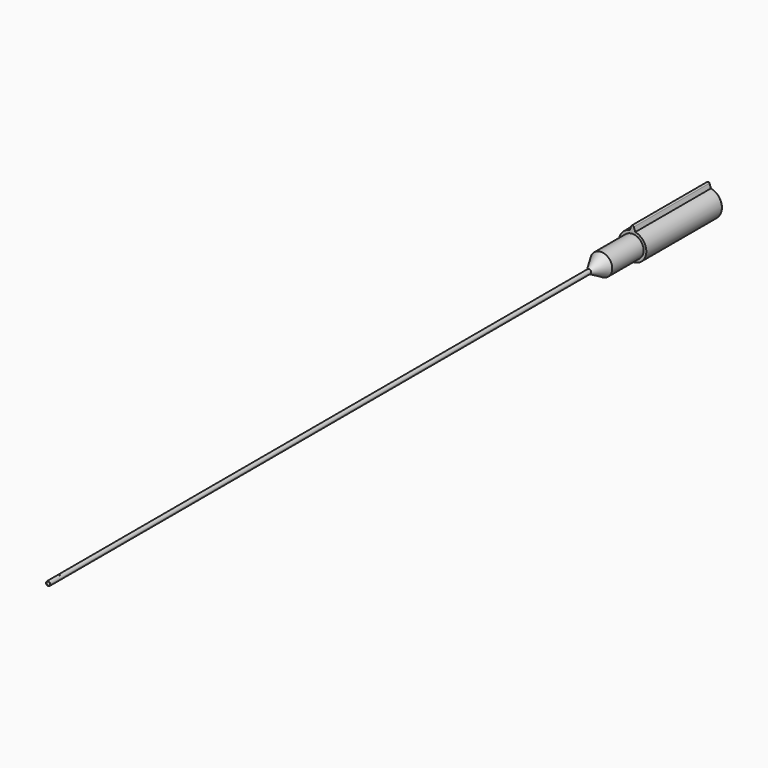
from build123d import *

# Parameters (mm, degrees)
F0_R     = 0.8
F0_R_2   = 0.66
F1_DEPTH = 248
F2_R     = 0.25
F3_DEPTH = 1
F7_R     = 4.040390162
F8_DEPTH = 5
F9_DEPTH = 35
F10_R    = 0.49999


# Not quite as in the source:
# - a fillet or chamfer is up to 0.001 mm smaller than in the source, because OpenCascade refuses the exact size


with BuildPart() as f1:
    # F0 (on Front) → F1 (new body)
    with BuildSketch(Plane.XZ):
        Circle(F0_R)
        Circle(F0_R_2, mode=Mode.SUBTRACT)
    extrude(amount=-F1_DEPTH)

    # F2 (on Top) → F3 (cut)
    with BuildSketch(Plane.XY):
        with Locations((0, 5)):
            Circle(F2_R)
    extrude(amount=F3_DEPTH, mode=Mode.SUBTRACT)


with BuildPart() as f5:
    # F4 (on Right) → F5 (revolve)
    with BuildSketch(Plane.YZ):
        Polygon((253.6107184147, 4.040390162), (247.9884784147, 0.7943883846), (247.9884784147, 0.6517949142), (302.9887184147, 0.6517949142), (302.9887184147, 5.040390162), (267.9887184147, 5.040390162), (267.9887184147, 4.040390162), align=None)
    revolve(axis=Axis((0, 127.867102623, 0), (0, 1, 0)))

    # F7 (on offset) → F8 (cut)
    with BuildSketch(Plane(origin=(0, 302.9887184147, 0), x_dir=(-1, 0, 0), z_dir=(0, 1, 0))):
        Circle(F7_R)
    extrude(amount=-F8_DEPTH, mode=Mode.SUBTRACT)

    # F7 (on offset) → F9 (join)
    with BuildSketch(Plane(origin=(0, 302.9887184147, 0), x_dir=(-1, 0, 0), z_dir=(0, 1, 0))):
        Polygon((0, 7.7686227672), (-1, 4.9401956424), (1, 4.9401956424), align=None)
    extrude(amount=-F9_DEPTH)

    # F10 (radius 0.5 in the source; OpenCascade refuses exactly that, so slightly less here)
    f10_edges = [f5.edges().sort_by_distance(p)[0] for p in [
        (0, 302.988718, -5.04039),
        (4.04039, 302.988718, 0),
        (4.04039, 297.988718, 0),
        (0, 297.988718, -0.651795),
        (0.5, 302.988718, 6.354409),
        (-0.5, 302.988718, 6.354409),
        (0, 285.488718, 7.768623),
    ]]
    fillet(f10_edges, radius=F10_R)


solid = Compound([f1.part, f5.part])
